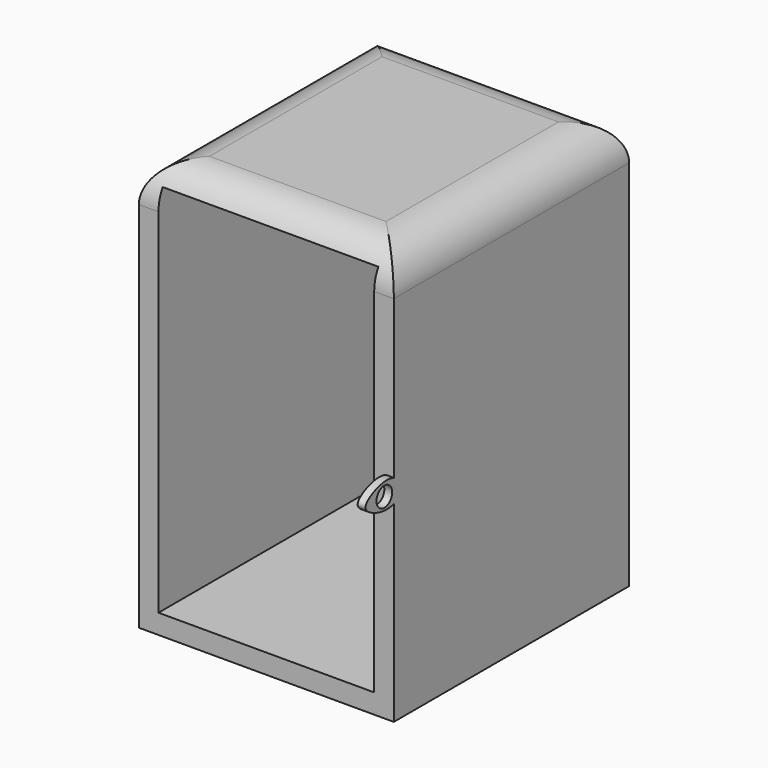
from build123d import *

# Parameters (mm, degrees)
F0_W        = 330.2
F0_H        = 533.4
F0_W_2      = 279.4
F0_H_2      = 482.6
F1_DEPTH    = 381
F2_R        = 12.7
F3_DEPTH    = 10.16
F4_T1_DEPTH = 635
F4_T3_DEPTH = 584.2


# Not quite as in the source:
# - a fillet or chamfer that OpenCascade refuses, or shapes differently, is made with other operations: its cross-section is extruded or revolved along the edge and cut away or added


with BuildPart() as f1:
    # F0 (on Front) → F1 (new body)
    with BuildSketch(Plane.XZ):
        Rectangle(F0_W, F0_H)
        Rectangle(F0_W_2, F0_H_2, mode=Mode.SUBTRACT)
    extrude(amount=F1_DEPTH)

    # F2 (on face) → F3 (join)
    with BuildSketch(Plane.YZ.offset(165.1)):
        with BuildLine():
            add(Edge.make_bspline(
                [(-378.2229094568, 10.4518691667), (-385.9598838993, 14.4257039209), (-405.6146401633, 14.5371341372), (-437.0263849997, -3.7421973966), (-405.4977582368, -20.7209483443), (-378.1421616626, -20.5633411646), (-363.038665815, -3.6640736551), (-372.1410397823, 7.3281228932), (-378.2229094568, 10.4518691667)],
                knots=[0, 0, 0, 0, 0.1843978335, 0.3570613059, 0.5281889509, 0.7125867844, 0.8550488179, 1, 1, 1, 1], degree=3))
        make_face()
        with Locations((-396.3470816139, -3.5818209283)):
            Circle(F2_R, mode=Mode.SUBTRACT)
    extrude(amount=-F3_DEPTH)

    # F4: fillet of radius 50.8 on 4 edges, made by hand

    # F4_s2 → F4_t1 (cut)
    with BuildSketch(Plane.XZ.offset(-127)):
        with BuildLine():
            ThreePointArc((165.1, 215.9), (150.2210244843, 251.8210244843), (114.3, 266.7))
            Line((114.3, 266.7), (165.1, 266.7))
            Line((165.1, 266.7), (165.1, 215.9))
        make_face()
        with BuildLine():
            ThreePointArc((-165.1, 215.9), (-150.2210244843, 251.8210244843), (-114.3, 266.7))
            Line((-114.3, 266.7), (-165.1, 266.7))
            Line((-165.1, 266.7), (-165.1, 215.9))
        make_face()
    extrude(amount=F4_T1_DEPTH, mode=Mode.SUBTRACT)

    # F4_s4 → F4_t3 (cut)
    with BuildSketch(Plane.YZ.offset(-292.1)):
        with BuildLine():
            ThreePointArc((0, 215.9), (-14.8789755157, 251.8210244843), (-50.8, 266.7))
            Line((-50.8, 266.7), (0, 266.7))
            Line((0, 266.7), (0, 215.9))
        make_face()
        with BuildLine():
            ThreePointArc((-381, 215.9), (-366.1210244843, 251.8210244843), (-330.2, 266.7))
            Line((-330.2, 266.7), (-381, 266.7))
            Line((-381, 266.7), (-381, 215.9))
        make_face()
    extrude(amount=F4_T3_DEPTH, mode=Mode.SUBTRACT)


solid = f1.part
